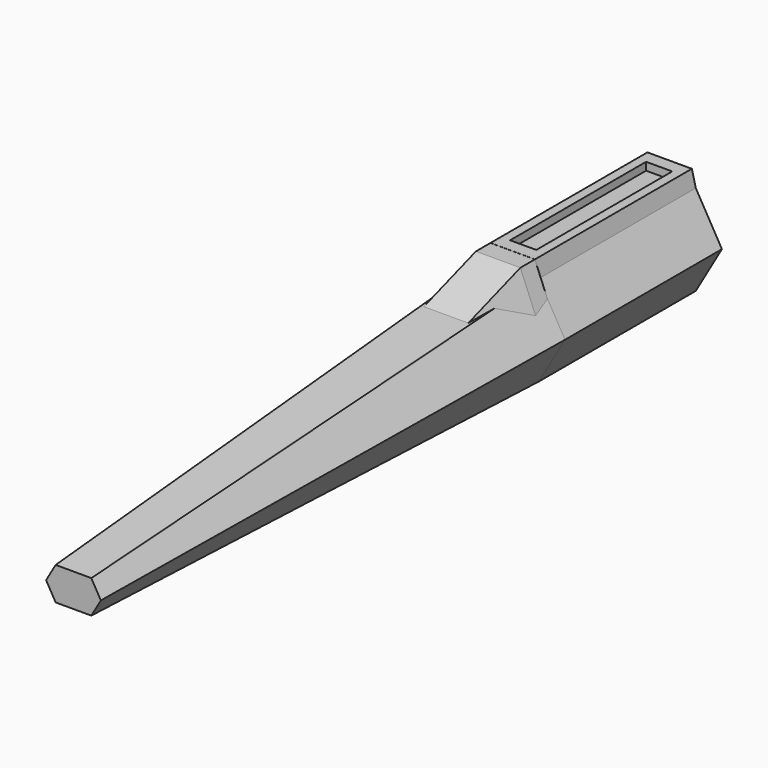
from build123d import *

# Parameters (mm, degrees)
F1_DEPTH  = 75
F3_DEPTH  = 210
F3_TAPER  = 1.5
F7_DEPTH  = 75
F10_W     = 10
F10_H     = 3
F11_DEPTH = 65


# Not quite as in the source:
# - a feature names something its author has since deleted; it is built from what else it names


with BuildPart() as f1:
    # F0 (on Front) → F1 (new body)
    with BuildSketch(Plane.XZ):
        Polygon((-10, -17.3205080757), (10, -17.3205080757), (20, 0), (10, 17.3205080757), (-10, 17.3205080757), (-20, 0), align=None)
    extrude(amount=-F1_DEPTH)

    # F2 (on face) → F3 (join)
    with BuildSketch(Plane.XZ):
        Polygon((10, -17.3205080757), (20, 0), (-20, 0), (-10, -17.3205080757), align=None)
    extrude(amount=F3_DEPTH, taper=F3_TAPER)

    # F4 (on face) → F6 section 0
    with BuildSketch(Plane.XZ.offset(210)):
        Polygon((-10.4753772138, -5.4990435295), (10.4753772138, -5.4990435295), (6.8251257379, 0.8233774871), (-6.8251257379, 0.8233774871), align=None)
    # F5 (on face) → F6 section 1
    with BuildSketch(Plane.XZ):
        Polygon((-10, 17.3205080757), (-20, 0), (20, 0), (10, 17.3205080757), align=None)
    loft()

    # F0 (on Front) → F7 (join, through all)
    with BuildSketch(Plane.XZ):
        Polygon((-10, 17.3205080757), (10, 17.3205080757), (8.5, 23.3205080757), (-8.5, 23.3205080757), align=None)
    extrude(amount=-F7_DEPTH)

    # F10 (on offset) → F11 (cut)
    with BuildSketch(Plane.XZ.offset(-5)):
        with Locations((0, 21.8205080757)):
            Rectangle(F10_W, F10_H)
    extrude(amount=-F11_DEPTH, mode=Mode.SUBTRACT)

    # F14: sweep along a path in F13
    with BuildLine(Plane.YZ) as f14_path:
        Line((-7.1518244222, 23.3403816819), (-35.0594446063, 13.796761632))
    # F12 (on offset) → F14 (sweep)
    with BuildSketch(Plane.XZ.offset(7)):
        Polygon((-8.5, 23.3205080757), (-15.4033075124, 4.9551053697), (16.0198838661, 4.9551053697), (8.5, 23.3205080757), align=None)
    sweep(path=f14_path.line)

    # F16: sweep along a path in F15
    with BuildLine(Plane.YZ) as f16_path:
        Line((-6.9480864331, 23.3692936599), (0, 23.3692936599))
    # F12 (on offset) → F16 (sweep)
    with BuildSketch(Plane.XZ.offset(7)):
        Polygon((-8.5, 23.3205080757), (-15.4033075124, 4.9551053697), (16.0198838661, 4.9551053697), (8.5, 23.3205080757), align=None)
    sweep(path=f16_path.line)


solid = f1.part
